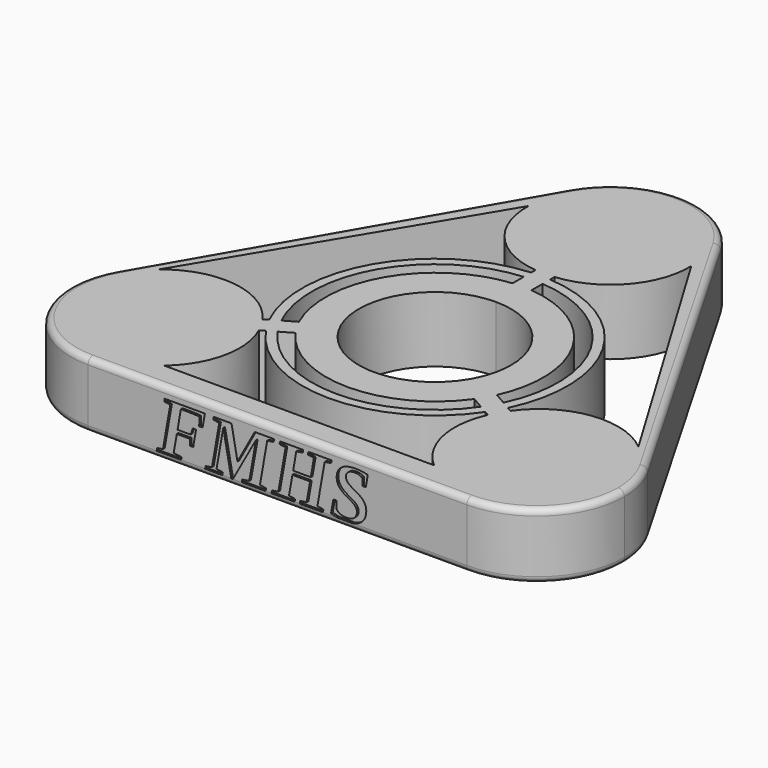
from build123d import *

# Parameters (mm, degrees)
F1_DEPTH  = 9.525
F3_DEPTH  = 25.4
F4_R      = 0.889
F6_DEPTH  = 0.3048
F8_DEPTH  = 25.4
F9_DEPTH  = 25.4
F10_R     = 11.049
F11_DEPTH = 9.525


with BuildPart() as f1:
    # F0 (on Top) → F1 (new body)
    with BuildSketch(Plane.XY):
        with BuildLine():
            ThreePointArc((-14.7963065702, -15.875), (-15.2290485763, -12.5879981272), (-16.4977839421, -9.525))
            ThreePointArc((-16.4977839421, -9.525), (-27.4963065702, -3.175), (-38.4948291982, -9.525))
            ThreePointArc((-38.4948291982, -9.525), (-38.4948291982, -22.225), (-27.4963065702, -28.575))
            ThreePointArc((-27.4963065702, -28.575), (-18.5160504491, -24.8552561211), (-14.7963065702, -15.875))
        make_face()
        with BuildLine():
            ThreePointArc((-16.4473065702, -15.875), (-38.1688210248, -18.7346916293), (-17.9275918837, -10.3505))
            ThreePointArc((-17.9275918837, -10.3505), (-16.8237921155, -13.0153083707), (-16.4473065702, -15.875))
        make_face(mode=Mode.SUBTRACT)
        with BuildLine():
            ThreePointArc((-10.9985226281, 38.1), (-10.9985226281, 25.4), (0, 19.05))
            ThreePointArc((0, 19.05), (8.9802561211, 22.7697438789), (12.7, 31.75))
            ThreePointArc((12.7, 31.75), (12.2672579939, 35.0370018728), (10.9985226281, 38.1))
            ThreePointArc((10.9985226281, 38.1), (0, 44.45), (-10.9985226281, 38.1))
        make_face()
        with BuildLine():
            ThreePointArc((11.049, 31.75), (7.8128228253, 23.9371771747), (0, 20.701))
            ThreePointArc((0, 20.701), (-7.8128228253, 39.5628228253), (11.049, 31.75))
        make_face(mode=Mode.SUBTRACT)
        with BuildLine():
            ThreePointArc((38.4948291982, -9.525), (27.4963065702, -3.175), (16.4977839421, -9.525))
            ThreePointArc((16.4977839421, -9.525), (16.4977839421, -22.225), (27.4963065702, -28.575))
            ThreePointArc((27.4963065702, -28.575), (36.4765626912, -24.8552561211), (40.1963065702, -15.875))
            ThreePointArc((40.1963065702, -15.875), (39.763564564, -12.5879981272), (38.4948291982, -9.525))
        make_face()
        with BuildLine():
            ThreePointArc((38.5453065702, -15.875), (24.6366149408, -26.5475144547), (17.9275918837, -10.3505))
            ThreePointArc((17.9275918837, -10.3505), (30.3559981995, -5.2024855453), (38.5453065702, -15.875))
        make_face(mode=Mode.SUBTRACT)
        with BuildLine():
            ThreePointArc((10.9985226281, -6.35), (12.2672579939, -3.2870018728), (12.7, 0))
            ThreePointArc((12.7, 0), (8.9802561211, 8.9802561211), (0, 12.7))
            Line((0, 12.7), (0, 11.049))
            ThreePointArc((0, 11.049), (7.8128228253, 7.8128228253), (11.049, 0))
            ThreePointArc((11.049, 0), (10.6725144547, -2.8596916293), (9.5687146864, -5.5245))
            Line((9.5687146864, -5.5245), (10.9985226281, -6.35))
        make_face()
        with BuildLine():
            Line((0, 11.049), (0, 12.7))
            ThreePointArc((0, 12.7), (-10.9985226281, 6.35), (-10.9985226281, -6.35))
            Line((-10.9985226281, -6.35), (-9.5687146864, -5.5245))
            ThreePointArc((-9.5687146864, -5.5245), (-9.5687146864, 5.5245), (0, 11.049))
        make_face()
        with BuildLine():
            ThreePointArc((-10.9985226281, -6.35), (0, -12.7), (10.9985226281, -6.35))
            Line((10.9985226281, -6.35), (9.5687146864, -5.5245))
            ThreePointArc((9.5687146864, -5.5245), (0, -11.049), (-9.5687146864, -5.5245))
            Line((-9.5687146864, -5.5245), (-10.9985226281, -6.35))
        make_face()
        with BuildLine():
            ThreePointArc((-10.9985226281, -6.35), (-10.9985226281, 6.35), (0, 12.7))
            Line((0, 12.7), (0, 19.05))
            ThreePointArc((0, 19.05), (-10.9985226281, 25.4), (-10.9985226281, 38.1))
            Line((-10.9985226281, 38.1), (-38.4948291982, -9.525))
            ThreePointArc((-38.4948291982, -9.525), (-27.4963065702, -3.175), (-16.4977839421, -9.525))
            Line((-16.4977839421, -9.525), (-10.9985226281, -6.35))
        make_face()
        with BuildLine():
            Line((16.4977839421, -9.525), (10.9985226281, -6.35))
            ThreePointArc((10.9985226281, -6.35), (0, -12.7), (-10.9985226281, -6.35))
            Line((-10.9985226281, -6.35), (-16.4977839421, -9.525))
            ThreePointArc((-16.4977839421, -9.525), (-15.2290485763, -12.5879981272), (-14.7963065702, -15.875))
            ThreePointArc((-14.7963065702, -15.875), (-18.5160504491, -24.8552561211), (-27.4963065702, -28.575))
            Line((-27.4963065702, -28.575), (27.4963065702, -28.575))
            ThreePointArc((27.4963065702, -28.575), (16.4977839421, -22.225), (16.4977839421, -9.525))
        make_face()
        with BuildLine():
            ThreePointArc((0, 12.7), (8.9802561211, 8.9802561211), (12.7, 0))
            ThreePointArc((12.7, 0), (12.2672579939, -3.2870018728), (10.9985226281, -6.35))
            Line((10.9985226281, -6.35), (16.4977839421, -9.525))
            ThreePointArc((16.4977839421, -9.525), (27.4963065702, -3.175), (38.4948291982, -9.525))
            Line((38.4948291982, -9.525), (10.9985226281, 38.1))
            ThreePointArc((10.9985226281, 38.1), (12.2672579939, 35.0370018728), (12.7, 31.75))
            ThreePointArc((12.7, 31.75), (8.9802561211, 22.7697438789), (0, 19.05))
            Line((0, 19.05), (0, 12.7))
        make_face()
    extrude(amount=F1_DEPTH)

    # F2 (on face) → F3 (cut)
    with BuildSketch(Plane.XY.offset(9.525)):
        with BuildLine():
            Line((1.3716, 17.8289184192), (1.3716, 15.8009815823))
            ThreePointArc((1.3716, 15.8009815823), (13.6618125012, 7.8876511252), (14.369851455, -6.7126503473))
            Line((14.369851455, -6.7126503473), (16.1260962731, -7.7266187658))
            ThreePointArc((16.1260962731, -7.7266187658), (15.4859198603, 8.9408), (1.3716, 17.8289184192))
        make_face()
        with BuildLine():
            ThreePointArc((12.998251455, -9.088331235), (0, -15.7753022503), (-12.998251455, -9.088331235))
            Line((-12.998251455, -9.088331235), (-14.7544962731, -10.1022996535))
            ThreePointArc((-14.7544962731, -10.1022996535), (0, -17.8816), (14.7544962731, -10.1022996535))
            Line((14.7544962731, -10.1022996535), (12.998251455, -9.088331235))
        make_face()
        with BuildLine():
            ThreePointArc((-14.369851455, -6.7126503473), (-13.6618125012, 7.8876511252), (-1.3716, 15.8009815823))
            Line((-1.3716, 15.8009815823), (-1.3716, 17.8289184192))
            ThreePointArc((-1.3716, 17.8289184192), (-15.4859198603, 8.9408), (-16.1260962731, -7.7266187658))
            Line((-16.1260962731, -7.7266187658), (-14.369851455, -6.7126503473))
        make_face()
    extrude(amount=-F3_DEPTH, mode=Mode.SUBTRACT)

    # F4
    f4_edges = [f1.edges().sort_by_distance(p)[0] for p in [
        (-24.746676, 14.2875, 9.525),
        (-38.494829, -9.525, 4.7625),
        (-27.496307, -28.575, 4.7625),
        (-38.494829, -22.225, 0),
        (-38.494829, -22.225, 9.525),
        (27.496307, -28.575, 4.7625),
        (0, -28.575, 0),
        (0, -28.575, 9.525),
        (38.494829, -9.525, 4.7625),
        (38.494829, -22.225, 0),
        (38.494829, -22.225, 9.525),
        (10.998523, 38.1, 4.7625),
        (24.746676, 14.2875, 0),
        (24.746676, 14.2875, 9.525),
        (-10.998523, 38.1, 4.7625),
        (0, 44.45, 0),
        (0, 44.45, 9.525),
    ]]
    fillet(f4_edges, radius=F4_R)

    # F5 (on face) → F6 (cut)
    with BuildSketch(Plane.XZ.offset(28.575)):
        with BuildLine():
            Line((-15.0709742915, 1.4152176649), (-14.613686097, 3.9992322049))
            Line((-14.613686097, 3.9992322049), (-12.7071978158, 3.9992322049))
            Line((-12.7071978158, 3.9992322049), (-12.702154196, 3.0964242622))
            Line((-12.702154196, 3.0964242622), (-12.2347787619, 3.0964242622))
            Line((-12.2347787619, 3.0964242622), (-11.8144771126, 5.4702879774))
            Line((-11.8144771126, 5.4702879774), (-12.2818525467, 5.4702879774))
            Line((-12.2818525467, 5.4702879774), (-12.6029630067, 4.5775672743))
            Line((-12.6029630067, 4.5775672743), (-14.509451288, 4.5775672743))
            Line((-14.509451288, 4.5775672743), (-14.0202201682, 7.3566017795))
            Line((-14.0202201682, 7.3566017795), (-13.2956201248, 7.3566017795))
            add(Edge.make_bspline(
                [(-12.2423441916, 7.3381085069), (-12.9123050206, 7.3566017795), (-13.2956201248, 7.3566017795)],
                knots=[0, 0, 0, 1, 1, 1], degree=2))
            add(Edge.make_bspline(
                [(-11.3151587533, 7.2826286892), (-11.5723833626, 7.3196152344), (-12.2423441916, 7.3381085069)],
                knots=[0, 0, 0, 1, 1, 1], degree=2))
            Line((-11.3151587533, 7.2826286892), (-11.3672761578, 6.0385358073))
            Line((-11.3672761578, 6.0385358073), (-10.8730014182, 6.0385358073))
            Line((-10.8730014182, 6.0385358073), (-10.5367600987, 7.934936849))
            Line((-10.5367600987, 7.934936849), (-16.3739094043, 7.934936849))
            Line((-16.3739094043, 7.934936849), (-16.4428388748, 7.5516217448))
            Line((-16.4428388748, 7.5516217448), (-15.565249031, 7.4137628038))
            Line((-15.565249031, 7.4137628038), (-16.6210467741, 1.4152176649))
            Line((-16.6210467741, 1.4152176649), (-17.4835057585, 1.2723151042))
            Line((-17.4835057585, 1.2723151042), (-17.5457104026, 0.889))
            Line((-17.5457104026, 0.889), (-13.9899584494, 0.889))
            Line((-13.9899584494, 0.889), (-13.9260725987, 1.2723151042))
            Line((-13.9260725987, 1.2723151042), (-15.0709742915, 1.4152176649))
        make_face()
        Polygon((-10.4375689095, 1.2723151042), (-10.4997735536, 0.889), (-7.9947757237, 0.889), (-7.9308898731, 1.2723151042), (-8.8505098817, 1.4152176649), (-7.868685229, 6.9732866753), (-6.7069714703, 0.889), (-6.4699213401, 0.889), (-3.114232972, 6.9732866753), (-4.0960576248, 1.4152176649), (-5.1199124425, 1.2723151042), (-5.1837982932, 0.889), (-1.7322811491, 0.889), (-1.6683952984, 1.2723151042), (-2.5459851422, 1.4152176649), (-1.4901873991, 7.4137628038), (-0.5604801508, 7.5516217448), (-0.4915506803, 7.934936849), (-3.3025281109, 7.934936849), (-5.8041635276, 3.3418804253), (-6.6699849251, 7.934936849), (-9.2607242915, 7.934936849), (-9.3279725553, 7.5516217448), (-8.4520639182, 7.4137628038), (-9.5078616612, 1.4152176649), align=None)
        Polygon((-0.8008926942, 1.277358724), (-0.8698221647, 0.889), (2.4825037901, 0.889), (2.5514332606, 1.277358724), (1.6738434169, 1.4152176649), (2.1664369499, 4.2245138889), (4.7302770106, 4.2245138889), (4.2376834776, 1.4152176649), (3.3079762294, 1.277358724), (3.2390467589, 0.889), (6.6065035731, 0.889), (6.6754330436, 1.277358724), (5.7927995801, 1.4152176649), (6.8485973231, 7.408719184), (7.7833481912, 7.5516217448), (7.8522776617, 7.934936849), (4.4848208474, 7.934936849), (4.4158913769, 7.5516217448), (5.2934812207, 7.408719184), (4.8361930263, 4.8028489583), (2.2723529655, 4.8028489583), (2.7296411599, 7.408719184), (3.6593484082, 7.5516217448), (3.7282778787, 7.934936849), (0.370908304, 7.934936849), (0.3019788335, 7.5516217448), (1.1795686773, 7.408719184), (0.1237709342, 1.4152176649), align=None)
        with BuildLine():
            Line((8.6916401873, 0.889), (10.9713653598, 0.889))
            add(Edge.make_bspline(
                [(12.1090927658, 1.3799123264), (11.6576337923, 1.0345072928), (10.9713653598, 0.889)],
                knots=[0, 0, 0, 0.5787343015, 0.5787343015, 0.5787343015], degree=2))
            add(Edge.make_bspline(
                [(12.8891726269, 3.1115551215), (12.8891726269, 1.9767406684), (12.1090927658, 1.3799123264)],
                knots=[0, 0, 0, 1, 1, 1], degree=2))
            add(Edge.make_bspline(
                [(12.7605603223, 3.8100964627), (12.8891726269, 3.5100010851), (12.8891726269, 3.1115551215)],
                knots=[0, 0, 0, 1, 1, 1], degree=2))
            add(Edge.make_bspline(
                [(12.4167535731, 4.3464013672), (12.6319480176, 4.1101918403), (12.7605603223, 3.8100964627)],
                knots=[0, 0, 0, 1, 1, 1], degree=2))
            add(Edge.make_bspline(
                [(11.8888547016, 4.7902399089), (12.2015591287, 4.5826108941), (12.4167535731, 4.3464013672)],
                knots=[0, 0, 0, 1, 1, 1], degree=2))
            add(Edge.make_bspline(
                [(10.8717247103, 5.3912712674), (11.5761502745, 4.9978689236), (11.8888547016, 4.7902399089)],
                knots=[0, 0, 0, 1, 1, 1], degree=2))
            add(Edge.make_bspline(
                [(10.1605743197, 5.925054362), (10.3892184169, 5.6602643229), (10.8717247103, 5.3912712674)],
                knots=[0, 0, 0, 1, 1, 1], degree=2))
            add(Edge.make_bspline(
                [(9.9319302224, 6.5059112413), (9.9319302224, 6.189844401), (10.1605743197, 5.925054362)],
                knots=[0, 0, 0, 1, 1, 1], degree=2))
            add(Edge.make_bspline(
                [(10.2706933518, 7.2094962023), (9.9319302224, 6.9514309896), (9.9319302224, 6.5059112413)],
                knots=[0, 0, 0, 1, 1, 1], degree=2))
            add(Edge.make_bspline(
                [(11.2029224099, 7.4675614149), (10.6094564811, 7.4675614149), (10.2706933518, 7.2094962023)],
                knots=[0, 0, 0, 1, 1, 1], degree=2))
            add(Edge.make_bspline(
                [(12.3125187641, 7.1414073351), (11.887173495, 7.4675614149), (11.2029224099, 7.4675614149)],
                knots=[0, 0, 0, 1, 1, 1], degree=2))
            Line((12.3125187641, 7.1414073351), (12.3495053092, 6.110827691))
            Line((12.3495053092, 6.110827691), (12.8168807433, 6.110827691))
            Line((12.8168807433, 6.110827691), (13.1110918978, 7.7869906684))
            add(Edge.make_bspline(
                [(11.3458249707, 8.013953559), (12.2435892936, 8.013953559), (13.1110918978, 7.7869906684)],
                knots=[0, 0, 0, 1, 1, 1], degree=2))
            add(Edge.make_bspline(
                [(9.2989559386, 7.5062291667), (10.0008596929, 8.013953559), (11.3458249707, 8.013953559)],
                knots=[0, 0, 0, 1, 1, 1], degree=2))
            add(Edge.make_bspline(
                [(8.5970521842, 6.0318109809), (8.5970521842, 6.9985047743), (9.2989559386, 7.5062291667)],
                knots=[0, 0, 0, 1, 1, 1], degree=2))
            add(Edge.make_bspline(
                [(8.723142679, 5.3181387804), (8.5970521842, 5.6232777778), (8.5970521842, 6.0318109809)],
                knots=[0, 0, 0, 1, 1, 1], degree=2))
            add(Edge.make_bspline(
                [(9.0568621886, 4.7767902561), (8.8492331738, 5.012999783), (8.723142679, 5.3181387804)],
                knots=[0, 0, 0, 1, 1, 1], degree=2))
            add(Edge.make_bspline(
                [(9.5276000358, 4.3590104167), (9.2644912033, 4.5405807292), (9.0568621886, 4.7767902561)],
                knots=[0, 0, 0, 1, 1, 1], degree=2))
            add(Edge.make_bspline(
                [(10.0664267502, 4.0227690972), (9.7907088683, 4.1774401042), (9.5276000358, 4.3590104167)],
                knots=[0, 0, 0, 1, 1, 1], degree=2))
            add(Edge.make_bspline(
                [(10.6044128613, 3.7184707031), (10.3421446322, 3.8680980903), (10.0664267502, 4.0227690972)],
                knots=[0, 0, 0, 1, 1, 1], degree=2))
            add(Edge.make_bspline(
                [(11.0743101052, 3.3982008464), (10.8666810905, 3.568843316), (10.6044128613, 3.7184707031)],
                knots=[0, 0, 0, 1, 1, 1], degree=2))
            add(Edge.make_bspline(
                [(11.4080296148, 3.0174075521), (11.28193912, 3.2275583767), (11.0743101052, 3.3982008464)],
                knots=[0, 0, 0, 1, 1, 1], degree=2))
            add(Edge.make_bspline(
                [(11.5341201096, 2.5231328125), (11.5341201096, 2.8072567274), (11.4080296148, 3.0174075521)],
                knots=[0, 0, 0, 1, 1, 1], degree=2))
            add(Edge.make_bspline(
                [(11.1188620801, 1.6346151259), (11.5341201096, 1.9548849826), (11.5341201096, 2.5231328125)],
                knots=[0, 0, 0, 1, 1, 1], degree=2))
            add(Edge.make_bspline(
                [(9.9369738422, 1.3143452691), (10.7036040506, 1.3143452691), (11.1188620801, 1.6346151259)],
                knots=[0, 0, 0, 1, 1, 1], degree=2))
            add(Edge.make_bspline(
                [(9.1333570888, 1.4875095486), (9.5116285731, 1.3143452691), (9.9369738422, 1.3143452691)],
                knots=[0, 0, 0, 1, 1, 1], degree=2))
            add(Edge.make_bspline(
                [(8.5768777051, 1.9195796441), (8.7550856044, 1.6606738281), (9.1333570888, 1.4875095486)],
                knots=[0, 0, 0, 1, 1, 1], degree=2))
            Line((8.5768777051, 1.9195796441), (8.5718340853, 3.0476692708))
            Line((8.5718340853, 3.0476692708), (8.109502271, 3.0476692708))
            Line((8.109502271, 3.0476692708), (7.7732609516, 1.156311849))
            add(Edge.make_bspline(
                [(8.6916401873, 0.889), (8.210057316, 0.9819075452), (7.7732609516, 1.156311849)],
                knots=[0.5327136039, 0.5327136039, 0.5327136039, 1, 1, 1], degree=2))
        make_face()
    extrude(amount=-F6_DEPTH, mode=Mode.SUBTRACT)

    # F7 (on face) → F8 (cut)
    with BuildSketch(Plane.XY.offset(9.525)):
        with BuildLine():
            ThreePointArc((1.3716, 19.1705529419), (16.6740305377, 9.6124862327), (17.3236326551, -8.4180167183))
            Line((17.3236326551, -8.4180167183), (18.0055194088, -8.8117042192))
            ThreePointArc((18.0055194088, -8.8117042192), (25.9343705674, -4.0031599244), (34.8299739221, -6.6217511266))
            Line((34.8299739221, -6.6217511266), (11.811, 31.75))
            ThreePointArc((11.811, 31.75), (8.9247646407, 23.7948503638), (1.3716, 19.9785086347))
            Line((1.3716, 19.9785086347), (1.3716, 19.1705529419))
        make_face()
        with BuildLine():
            Line((-1.3716, 19.1705529419), (-1.3716, 19.9785086347))
            ThreePointArc((-1.3716, 19.9785086347), (-8.9247646407, 23.7948503638), (-11.811, 31.75))
            Line((-11.811, 31.75), (-34.8299739221, -6.6217511266))
            ThreePointArc((-34.8299739221, -6.6217511266), (-25.9343705674, -4.0031599244), (-18.0055194088, -8.8117042192))
            Line((-18.0055194088, -8.8117042192), (-17.3236326551, -8.4180167183))
            ThreePointArc((-17.3236326551, -8.4180167183), (-16.6740305377, 9.6124862327), (-1.3716, 19.1705529419))
        make_face()
    extrude(amount=-F8_DEPTH, mode=Mode.SUBTRACT)

    # F7 (on face) → F9 (cut)
    with BuildSketch(Plane.XY.offset(9.525)):
        with BuildLine():
            Line((16.6339194088, -11.1873851068), (15.9520326551, -10.793697606))
            ThreePointArc((15.9520326551, -10.793697606), (0.0123579978, -19.2463771455), (-15.9163858523, -10.7731169148))
            Line((-15.9163858523, -10.7731169148), (-16.6160960074, -11.1770947612))
            ThreePointArc((-16.6160960074, -11.1770947612), (-15.8534381423, -18.4072608372), (-19.586673065, -24.645842849))
            Line((-19.586673065, -24.645842849), (19.586673065, -24.645842849))
            ThreePointArc((19.586673065, -24.645842849), (15.8668933935, -18.4088112322), (16.6339194088, -11.1873851068))
        make_face()
    extrude(amount=-F9_DEPTH, mode=Mode.SUBTRACT)

    # F10 (on face) → F11 (join)
    with BuildSketch(Plane.XY.offset(9.525)):
        with Locations((0, 31.75)):
            Circle(F10_R)
        with Locations((27.4963065702, -15.875)):
            Circle(F10_R)
        with Locations((-27.4963065702, -15.875)):
            Circle(F10_R)
    extrude(amount=-F11_DEPTH)


solid = f1.part
